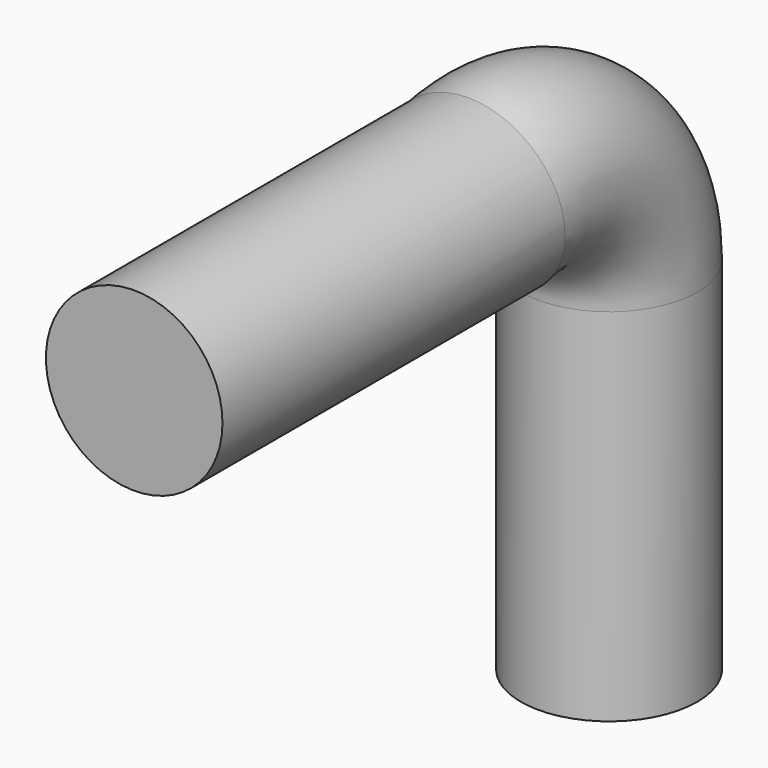
from build123d import *

# Parameters (mm, degrees)
F0_R = 8.627554


with BuildPart() as f2:
    # F2: sweep along a path in F1
    with BuildLine(Plane.YZ) as f2_path:
        Line((14.816666, 0), (14.816666, 35.244173))
        ThreePointArc((14.816666, 35.244173), (9.76363, 45.430051), (-1.403685, 47.569297))
        Line((-1.403685, 47.569297), (-43.202281, 47.569297))
    # F0 (on Top) → F2 (sweep)
    with BuildSketch(Plane.XY):
        with Locations((-34.624211, 14.816666)):
            Circle(F0_R)
    sweep(path=f2_path.line, transition=Transition.RIGHT)


solid = f2.part
